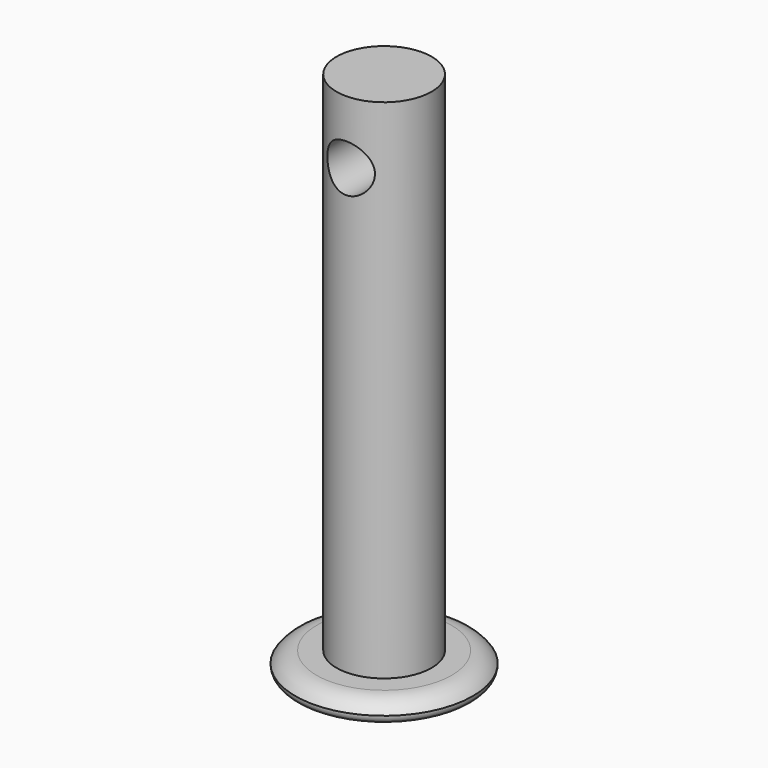
from build123d import *

# Parameters (mm, degrees)
F0_R     = 8.89
F1_DEPTH = 2.032
F2_R     = 4.76123
F3_DEPTH = 50.8
F5_DEPTH = 4.7625
F6_R     = 0.889


# Not quite as in the source:
# - a fillet or chamfer that OpenCascade refuses, or shapes differently, is made with other operations: its cross-section is extruded or revolved along the edge and cut away or added


with BuildPart() as f1:
    # F0 (on Top) → F1 (new body)
    with BuildSketch(Plane.XY):
        Circle(F0_R)
    extrude(amount=F1_DEPTH)

    # F2 (on face) → F3 (join)
    with BuildSketch(Plane.XY.offset(2.032)):
        Circle(F2_R)
    extrude(amount=F3_DEPTH)

    # F4 (on Front) → F5 (cut, symmetric)
    with BuildSketch(Plane.XZ):
        with BuildLine():
            ThreePointArc((0, 48.86325), (-1.6837980227, 44.7982019773), (2.38125, 46.482))
            ThreePointArc((2.38125, 46.482), (1.6837980227, 48.1657980227), (0, 48.86325))
        make_face()
    extrude(amount=F5_DEPTH, both=True, mode=Mode.SUBTRACT)

    # F6
    f6_edges = [f1.edges().sort_by_distance(p)[0] for p in [
        (-8.89, 0, 0),
    ]]
    fillet(f6_edges, radius=F6_R)

    # F7: fillet of radius 2.54 on 1 edges, made by hand

    # F7_s1 → F7_t2 (revolve, cut)
    with BuildSketch(Plane.XZ):
        with BuildLine():
            ThreePointArc((8.89, 0.889), (7.9735095663, 1.7280657414), (6.7686817778, 2.032))
            Line((6.7686817778, 2.032), (6.7686817778, 2.0828))
            Line((6.7686817778, 2.0828), (8.89, 2.0828))
            Line((8.89, 2.0828), (8.9408, 2.032))
            ThreePointArc((8.9408, 2.032), (8.9408, 1.4605), (8.9324263644, 0.91694))
            Line((8.9324263644, 0.91694), (8.89, 0.889))
        make_face()
    revolve(axis=Axis((0, 0, 2.032), (0, 0, 1)), mode=Mode.SUBTRACT)


solid = f1.part
